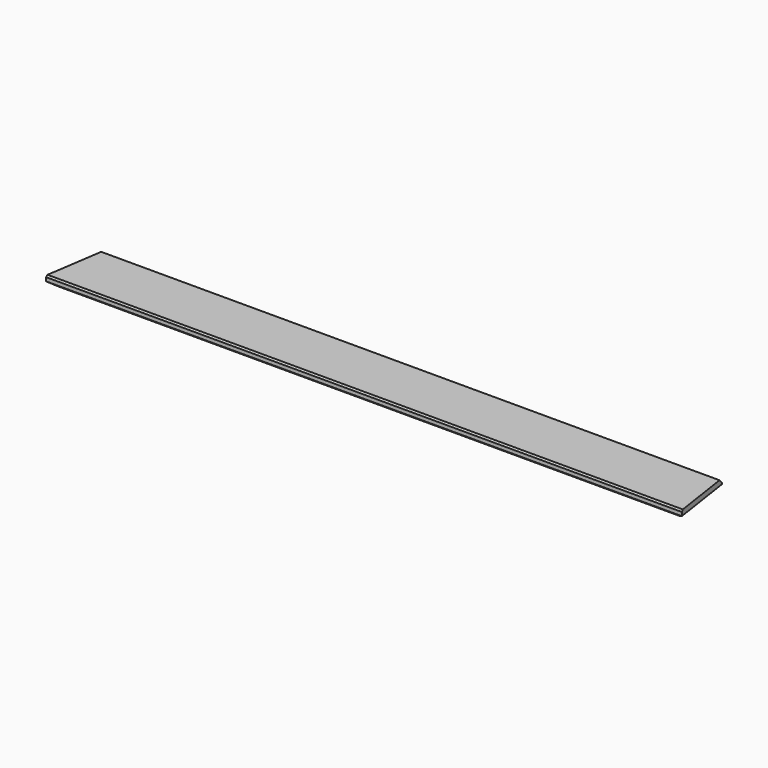
from build123d import *

# Parameters (mm, degrees)
F0_W      = 2000
F0_H      = 32
F1_DEPTH  = 200
F2_SIZE   = 12
F3_SIZE   = 5
F5_DEPTH  = 32
F6_SIZE   = 4.99999
F7_SIZE   = 4.99999
F9_DEPTH  = 2097
F10_SIZE2 = 15
F10_SIZE  = 20


# Not quite as in the source:
# - a fillet or chamfer is up to 0.001 mm smaller than in the source, because OpenCascade refuses the exact size


with BuildPart() as f1:
    # F0 (on Front) → F1 (new body)
    with BuildSketch(Plane.XZ):
        with Locations((-1000, 16)):
            Rectangle(F0_W, F0_H)
    extrude(amount=F1_DEPTH)

    # F2
    f2_edges = [f1.edges().sort_by_distance(p)[0] for p in [
        (-1000, 0, 32),
    ]]
    chamfer(f2_edges, length=F2_SIZE)

    # F3
    f3_edges = [f1.edges().sort_by_distance(p)[0] for p in [
        (-1000, -200, 32),
    ]]
    chamfer(f3_edges, length=F3_SIZE)

    # F4 (on Top) → F5 (join)
    with BuildSketch(Plane.XY):
        Polygon((30, -200), (0, 0), (0, -200), align=None)
        Polygon((-2000, 0), (-2030, -200), (-2000, -200), align=None)
    extrude(amount=F5_DEPTH)

    # F6 (size 5 in the source; OpenCascade refuses exactly that, so slightly less here)
    f6_edges = [f1.edges().sort_by_distance(p)[0] for p in [
        (-2015, -200, 32),
    ]]
    chamfer(f6_edges, length=F6_SIZE)

    # F7 (size 5 in the source; OpenCascade refuses exactly that, so slightly less here)
    f7_edges = [f1.edges().sort_by_distance(p)[0] for p in [
        (15, -200, 32),
    ]]
    chamfer(f7_edges, length=F7_SIZE)

    # F8 (on Right) → F9 (cut, symmetric)
    with BuildSketch(Plane.YZ):
        Polygon((-12, 32), (0, 20), (0, 32), align=None)
    extrude(amount=F9_DEPTH, both=True, mode=Mode.SUBTRACT)

    # F10
    f10_edges = [f1.edges().sort_by_distance(p)[0] for p in [
        (-1000, -200, 0),
        (-2015, -100, 0),
        (15, -100, 0),
    ]]
    f10_side = f1.faces().sort_by_distance((-1000, -100.492611, 0))[0]
    chamfer(f10_edges, length=F10_SIZE, length2=F10_SIZE2, reference=f10_side)


solid = f1.part
